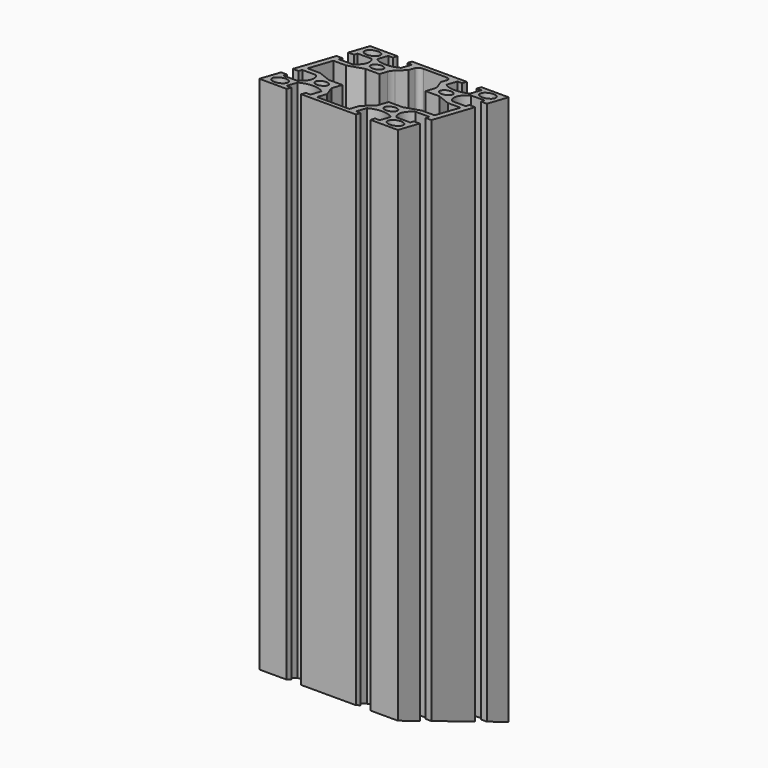
from build123d import *

# Parameters (mm, degrees)
F0_R          = 3
F0_R_2        = 2.5
F1_DEPTH      = 250
F2_R          = 2
F3_R          = 7
F5_DEPTH      = 30
F5_DEPTH_BACK = 30


# Not quite as in the source:
# - a feature names something its author has since deleted; it is built from what else it names


with BuildPart() as f1:
    # F0 (on Top) → F1 (new body)
    with BuildSketch(Plane.XY):
        with BuildLine():
            Line((18.15, -30), (30, -30))
            Line((30, -30), (30, -18.15))
            Line((30, -18.15), (27.5, -18.15))
            Line((27.5, -18.15), (27.5, -20.15))
            Line((27.5, -20.15), (21.5477069044, -20.15))
            ThreePointArc((21.5477069044, -20.15), (19.5, -15), (21.5477069044, -9.85))
            Line((21.5477069044, -9.85), (27.5, -9.85))
            Line((27.5, -9.85), (27.5, -11.85))
            Line((27.5, -11.85), (30, -11.85))
            Line((30, -11.85), (30, 11.85))
            Line((30, 11.85), (27.5, 11.85))
            Line((27.5, 11.85), (27.5, 9.85))
            Line((27.5, 9.85), (21.5477069044, 9.85))
            ThreePointArc((21.5477069044, 9.85), (19.5, 15), (21.5477069044, 20.15))
            Line((21.5477069044, 20.15), (27.5, 20.15))
            Line((27.5, 20.15), (27.5, 18.15))
            Line((27.5, 18.15), (30, 18.15))
            Line((30, 18.15), (30, 30))
            Line((30, 30), (18.15, 30))
            Line((18.15, 30), (18.15, 27.5))
            Line((18.15, 27.5), (20.15, 27.5))
            Line((20.15, 27.5), (20.15, 21.5477069044))
            ThreePointArc((20.15, 21.5477069044), (15, 19.5), (9.85, 21.5477069044))
            Line((9.85, 21.5477069044), (9.85, 27.5))
            Line((9.85, 27.5), (11.85, 27.5))
            Line((11.85, 27.5), (11.85, 30))
            Line((11.85, 30), (-11.85, 30))
            Line((-11.85, 30), (-11.85, 27.5))
            Line((-11.85, 27.5), (-9.85, 27.5))
            Line((-9.85, 27.5), (-9.85, 21.5477069044))
            ThreePointArc((-9.85, 21.5477069044), (-15, 19.5), (-20.15, 21.5477069044))
            Line((-20.15, 21.5477069044), (-20.15, 27.5))
            Line((-20.15, 27.5), (-18.15, 27.5))
            Line((-18.15, 27.5), (-18.15, 30))
            Line((-18.15, 30), (-30, 30))
            Line((-30, 30), (-30, 18.15))
            Line((-30, 18.15), (-27.5, 18.15))
            Line((-27.5, 18.15), (-27.5, 20.15))
            Line((-27.5, 20.15), (-21.5477069044, 20.15))
            ThreePointArc((-21.5477069044, 20.15), (-19.5, 15), (-21.5477069044, 9.85))
            Line((-21.5477069044, 9.85), (-27.5, 9.85))
            Line((-27.5, 9.85), (-27.5, 11.85))
            Line((-27.5, 11.85), (-30, 11.85))
            Line((-30, 11.85), (-30, -11.85))
            Line((-30, -11.85), (-27.5, -11.85))
            Line((-27.5, -11.85), (-27.5, -9.85))
            Line((-27.5, -9.85), (-21.5477069044, -9.85))
            ThreePointArc((-21.5477069044, -9.85), (-19.5, -15), (-21.5477069044, -20.15))
            Line((-21.5477069044, -20.15), (-27.5, -20.15))
            Line((-27.5, -20.15), (-27.5, -18.15))
            Line((-27.5, -18.15), (-30, -18.15))
            Line((-30, -18.15), (-30, -30))
            Line((-30, -30), (-18.15, -30))
            Line((-18.15, -30), (-18.15, -27.5))
            Line((-18.15, -27.5), (-20.15, -27.5))
            Line((-20.15, -27.5), (-20.15, -21.5477069044))
            ThreePointArc((-20.15, -21.5477069044), (-15, -19.5), (-9.85, -21.5477069044))
            Line((-9.85, -21.5477069044), (-9.85, -27.5))
            Line((-9.85, -27.5), (-11.85, -27.5))
            Line((-11.85, -27.5), (-11.85, -30))
            Line((-11.85, -30), (11.85, -30))
            Line((11.85, -30), (11.85, -27.5))
            Line((11.85, -27.5), (9.85, -27.5))
            Line((9.85, -27.5), (9.85, -21.5477069044))
            ThreePointArc((9.85, -21.5477069044), (15, -19.5), (20.15, -21.5477069044))
            Line((20.15, -21.5477069044), (20.15, -27.5))
            Line((20.15, -27.5), (18.15, -27.5))
            Line((18.15, -27.5), (18.15, -30))
        make_face()
        with Locations((-25, -25)):
            Circle(F0_R, mode=Mode.SUBTRACT)
        with Locations((-15, -15)):
            Circle(F0_R_2, mode=Mode.SUBTRACT)
        with Locations((25, -25)):
            Circle(F0_R, mode=Mode.SUBTRACT)
        with Locations((15, -15)):
            Circle(F0_R_2, mode=Mode.SUBTRACT)
        with Locations((-25, 25)):
            Circle(F0_R, mode=Mode.SUBTRACT)
        with Locations((-15, 15)):
            Circle(F0_R_2, mode=Mode.SUBTRACT)
        Polygon((-7, 22), (-7, 27.5), (0, 27.5), (7, 27.5), (7, 22), (10, 16), (10, 10), (16, 10), (22, 7), (27.5, 7), (27.5, 0), (27.5, -7), (22, -7), (16, -10), (10, -10), (10, -16), (7, -22), (7, -27.5), (0, -27.5), (-7, -27.5), (-7, -22), (-10, -16), (-10, -10), (-16, -10), (-22, -7), (-27.5, -7), (-27.5, 0), (-27.5, 7), (-22, 7), (-16, 10), (-10, 10), (-10, 16), align=None, mode=Mode.SUBTRACT)
        with Locations((15, 15)):
            Circle(F0_R_2, mode=Mode.SUBTRACT)
        with Locations((25, 25)):
            Circle(F0_R, mode=Mode.SUBTRACT)
    extrude(amount=F1_DEPTH)

    # F2
    f2_edges = [f1.edges().sort_by_distance(p)[0] for p in [
        (-7, 27.5, 125),
        (7, 27.5, 125),
    ]]
    fillet(f2_edges, radius=F2_R)

    # F3
    f3_edges = [f1.edges().sort_by_distance(p)[0] for p in [
        (-10, 16, 125),
        (10, 16, 125),
    ]]
    fillet(f3_edges, radius=F3_R)

    # F4 (on Right) → F5 (cut, two sides)
    with BuildSketch(Plane.YZ) as f5_sk:
        Polygon((-23.2563562234, -128.5722174771), (30, 0), (-168.5306378236, 82.2340827331), (-221.786994047, -46.338134744), align=None)
        Polygon((171.7491592878, 324.7994275924), (-8.0091289948, 360.5555742708), (-30, 250), (149.7582882826, 214.2438533216), align=None)
    extrude(amount=F5_DEPTH, mode=Mode.SUBTRACT)
    extrude(f5_sk.sketch, amount=-F5_DEPTH_BACK, mode=Mode.SUBTRACT)


solid = f1.part
